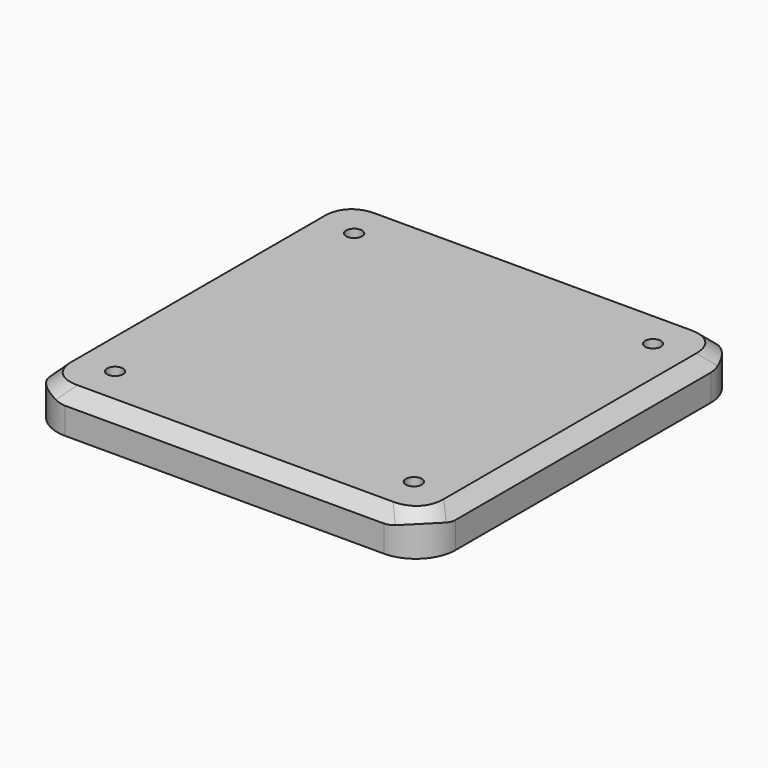
from build123d import *

# Parameters (mm, degrees)
F0_W     = 300
F0_H     = 300
F0_R     = 6
F1_DEPTH = 30
F2_DEPTH = 10
F3_DEPTH = 20
F4_SIZE2 = 10
F4_SIZE  = 10
F5_F1_R  = 30
F5_F2_R  = 30
F5_F3_R  = 30
F5_F4_R  = 30
F5_F5_R  = 30
F5_F6_R  = 30
F5_F7_R  = 30
F5_F8_R  = 30


with BuildPart() as f1:
    # F0 (on Top) → F1 (new body)
    with BuildSketch(Plane.XY):
        Rectangle(F0_W, F0_H)
        with Locations((-125, -125)):
            Circle(F0_R, mode=Mode.SUBTRACT)
        with Locations((-112.5, -112.5)):
            Circle(F0_R, mode=Mode.SUBTRACT)
        with Locations((125, -125)):
            Circle(F0_R, mode=Mode.SUBTRACT)
        with Locations((112.5, -112.5)):
            Circle(F0_R, mode=Mode.SUBTRACT)
        with Locations((-125, 125)):
            Circle(F0_R, mode=Mode.SUBTRACT)
        with Locations((-112.5, 112.5)):
            Circle(F0_R, mode=Mode.SUBTRACT)
        with Locations((112.5, 112.5)):
            Circle(F0_R, mode=Mode.SUBTRACT)
        with Locations((125, 125)):
            Circle(F0_R, mode=Mode.SUBTRACT)
        with Locations((-125, -125)):
            Circle(F0_R)
        with Locations((-125, 125)):
            Circle(F0_R)
        with Locations((125, 125)):
            Circle(F0_R)
        with Locations((125, -125)):
            Circle(F0_R)
    extrude(amount=F1_DEPTH)

    # F0 (on Top) → F2 (cut)
    with BuildSketch(Plane.XY):
        with Locations((-125, -125)):
            Circle(F0_R)
        with Locations((-125, 125)):
            Circle(F0_R)
        with Locations((125, 125)):
            Circle(F0_R)
        with Locations((125, -125)):
            Circle(F0_R)
    extrude(amount=F2_DEPTH, mode=Mode.SUBTRACT)

    # F0 (on Top) → F3 (join)
    with BuildSketch(Plane.XY):
        with Locations((-112.5, 112.5)):
            Circle(F0_R)
        with Locations((-112.5, -112.5)):
            Circle(F0_R)
        with Locations((112.5, 112.5)):
            Circle(F0_R)
        with Locations((112.5, -112.5)):
            Circle(F0_R)
    extrude(amount=F3_DEPTH)

    # F4
    f4_edges = [f1.edges().sort_by_distance(p)[0] for p in [
        (0, -150, 30),
        (-150, 0, 30),
        (150, 0, 30),
        (0, 150, 30),
    ]]
    chamfer(f4_edges, length=F4_SIZE, length2=F4_SIZE2)

    # F5: fillet of radius 30 on 8 edges, made by hand

    # F5_f1
    f5_f1_edges = [f1.edges().sort_by_distance(p)[0] for p in [
        (-150, -150, 10),
    ]]
    fillet(f5_f1_edges, radius=F5_F1_R)

    # F5_f2
    f5_f2_edges = [f1.edges().sort_by_distance(p)[0] for p in [
        (150, -150, 10),
    ]]
    fillet(f5_f2_edges, radius=F5_F2_R)

    # F5_f3
    f5_f3_edges = [f1.edges().sort_by_distance(p)[0] for p in [
        (-150, 150, 10),
    ]]
    fillet(f5_f3_edges, radius=F5_F3_R)

    # F5_f4
    f5_f4_edges = [f1.edges().sort_by_distance(p)[0] for p in [
        (-140.6066017178, -140.6066017178, 29.3933982822),
    ]]
    fillet(f5_f4_edges, radius=F5_F4_R)

    # F5_f5
    f5_f5_edges = [f1.edges().sort_by_distance(p)[0] for p in [
        (140.6066017178, -140.6066017178, 29.3933982822),
    ]]
    fillet(f5_f5_edges, radius=F5_F5_R)

    # F5_f6
    f5_f6_edges = [f1.edges().sort_by_distance(p)[0] for p in [
        (150, 150, 10),
    ]]
    fillet(f5_f6_edges, radius=F5_F6_R)

    # F5_f7
    f5_f7_edges = [f1.edges().sort_by_distance(p)[0] for p in [
        (-140.6066017178, 140.6066017178, 29.3933982822),
    ]]
    fillet(f5_f7_edges, radius=F5_F7_R)

    # F5_f8
    f5_f8_edges = [f1.edges().sort_by_distance(p)[0] for p in [
        (140.6066017178, 140.6066017178, 29.3933982822),
    ]]
    fillet(f5_f8_edges, radius=F5_F8_R)


solid = f1.part
